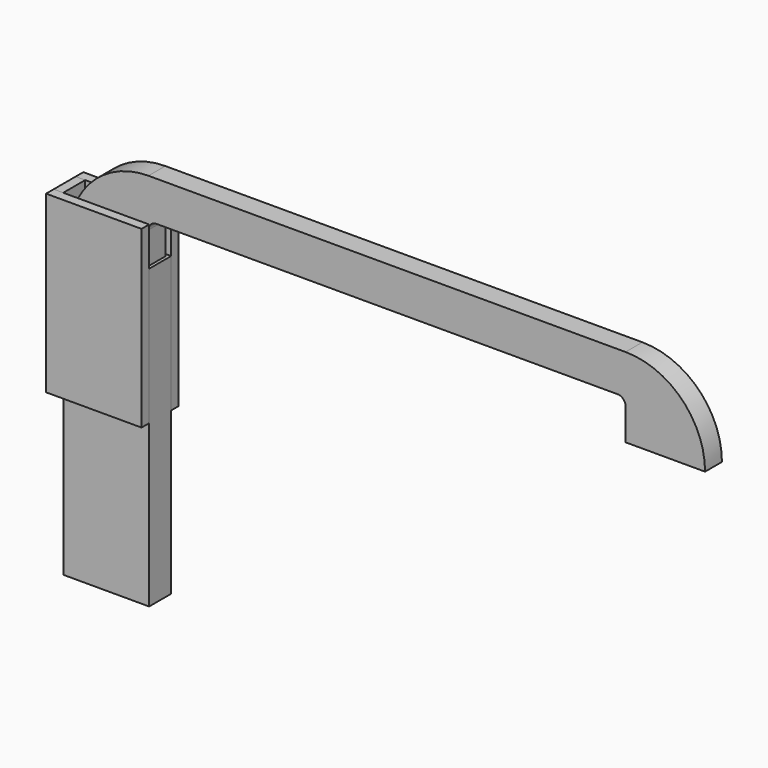
from build123d import *

# Parameters (mm, degrees)
F0_W          = 26.5
F0_H          = 100
F1_DEPTH      = 400
F1_DEPTH_BACK = 400
F2_W          = 600
F2_H          = 50
F3_DEPTH      = 26.501
F4_R          = 99.99999
F5_R          = 10
F6_W          = 108
F6_H          = 34.5
F6_W_2        = 100
F6_H_2        = 26.5
F7_DEPTH      = 374
F8_DEPTH      = 171
F8_DEPTH_BACK = 49
F6_W_3        = 12
F9_DEPTH      = 171
F9_DEPTH_BACK = 49


# Not quite as in the source:
# - a fillet or chamfer is up to 0.001 mm smaller than in the source, because OpenCascade refuses the exact size


with BuildPart() as f1:
    # F0 (on Right) → F1 (new body, two sides)
    with BuildSketch(Plane.YZ) as f1_sk:
        with Locations((-46.5, 40.5)):
            Rectangle(F0_W, F0_H)
    extrude(amount=F1_DEPTH)
    extrude(f1_sk.sketch, amount=-F1_DEPTH_BACK)

    # F2 (on face) → F3 (cut, through all)
    with BuildSketch(Plane.XZ.offset(59.75)):
        with Locations((0, 15.5)):
            Rectangle(F2_W, F2_H)
    extrude(amount=-F3_DEPTH, mode=Mode.SUBTRACT)

    # F4 (radius 100 in the source; OpenCascade refuses exactly that, so slightly less here)
    f4_edges = [f1.edges().sort_by_distance(p)[0] for p in [
        (-400, -46.5, 90.5),
        (400, -46.5, 90.5),
    ]]
    fillet(f4_edges, radius=F4_R)

    # F5
    f5_edges = [f1.edges().sort_by_distance(p)[0] for p in [
        (-300, -46.5, 40.5),
        (300, -46.5, 40.5),
    ]]
    fillet(f5_edges, radius=F5_R)


with BuildPart() as f7:
    # F6 (on face) → F7 (new body)
    with BuildSketch(Plane(origin=(0, 0, -9.5), x_dir=(1, 0, 0), z_dir=(0, 0, -1))):
        with Locations((-350, 46.5)):
            Rectangle(F6_W, F6_H)
        with Locations((-350, 46.5)):
            Rectangle(F6_W_2, F6_H_2, mode=Mode.SUBTRACT)
        with Locations((-350, 46.5)):
            Rectangle(F6_W_2, F6_H_2)
    extrude(amount=F7_DEPTH)


with BuildPart() as f8:
    # F6 (on face) → F8 (new body, two sides)
    with BuildSketch(Plane(origin=(0, 0, -9.5), x_dir=(1, 0, 0), z_dir=(0, 0, -1))) as f8_sk:
        Polygon((-404, 63.75), (-296, 63.75), (-296, 75.75), (-416, 75.75), (-416, 63.75), align=None)
    extrude(amount=F8_DEPTH)
    extrude(f8_sk.sketch, amount=-F8_DEPTH_BACK)


with BuildPart() as f8b:
    # F6 (on face) → F8, piece 2 (new body, two sides)
    with BuildSketch(Plane(origin=(0, 0, -9.5), x_dir=(1, 0, 0), z_dir=(0, 0, -1))) as f8_2_sk:
        Polygon((-296, 17.25), (-296, 29.25), (-404, 29.25), (-416, 29.25), (-416, 17.25), align=None)
    extrude(amount=F8_DEPTH)
    extrude(f8_2_sk.sketch, amount=-F8_DEPTH_BACK)


with BuildPart() as f9:
    # F6 (on face) → F9 (new body, two sides)
    with BuildSketch(Plane(origin=(0, 0, -9.5), x_dir=(1, 0, 0), z_dir=(0, 0, -1))) as f9_sk:
        with Locations((-410, 46.5)):
            Rectangle(F6_W_3, F6_H)
    extrude(amount=F9_DEPTH)
    extrude(f9_sk.sketch, amount=-F9_DEPTH_BACK)


solid = Compound([f1.part, f7.part, f8.part, f8b.part, f9.part])
